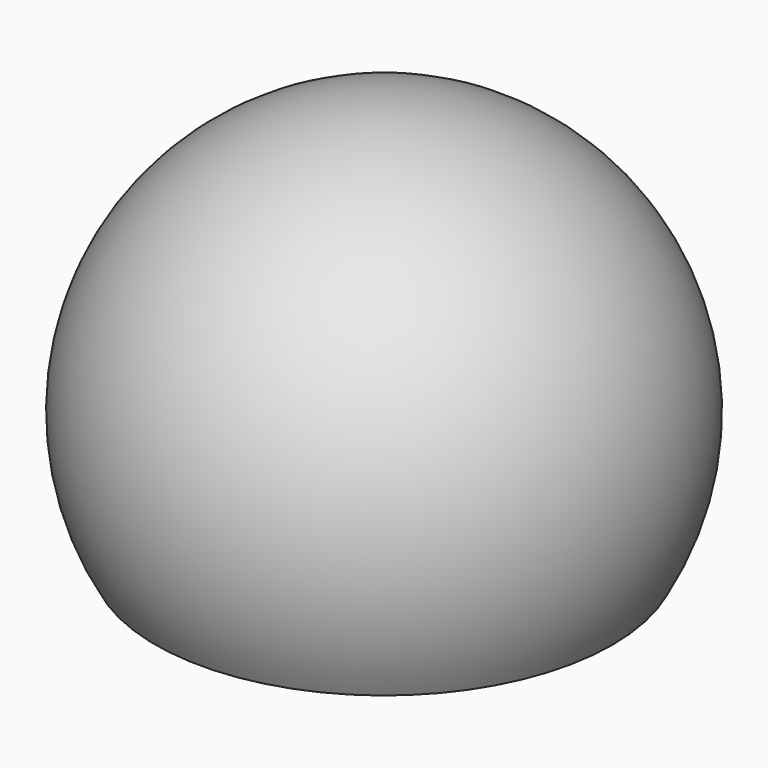
from build123d import *

# Parameters (mm, degrees)
F2_R = 1.19999
F3_R = 1.5


# Not quite as in the source:
# - a fillet or chamfer is up to 0.001 mm smaller than in the source, because OpenCascade refuses the exact size


with BuildPart() as f1:
    # F0 (on Front) → F1 (revolve)
    with BuildSketch(Plane.XZ):
        with BuildLine():
            Line((0, 22.8), (0, 24))
            ThreePointArc((0, 24), (-13.8564064606, 16), (-13.8564064606, 0))
            Line((-13.8564064606, 0), (-12.451505933, 0))
            ThreePointArc((-12.451505933, 0), (-13.8029789452, 13.3402033893), (-3.825, 22.2971806661))
            ThreePointArc((-3.825, 22.2971806661), (-3.227786159, 22.4437320839), (-2.625, 22.5653484339))
            ThreePointArc((-2.625, 22.5653484339), (-1.3177335047, 22.741220384), (0, 22.8))
        make_face()
        with BuildLine():
            Line((-2.625, 18.0653484339), (-2.625, 22.5653484339))
            ThreePointArc((-2.625, 22.5653484339), (-3.227786159, 22.4437320839), (-3.825, 22.2971806661))
            Line((-3.825, 22.2971806661), (-3.825, 18.0653484339))
            Line((-3.825, 18.0653484339), (-2.625, 18.0653484339))
        make_face()
    revolve(axis=Axis((0, 0, 23.4), (0, 0, 1)))

    # F2 (radius 1.2 in the source; OpenCascade refuses exactly that, so slightly less here)
    f2_edges = [f1.edges().sort_by_distance(p)[0] for p in [
        (2.625, 0, 18.065348),
    ]]
    fillet(f2_edges, radius=F2_R)

    # F3
    f3_edges = [f1.edges().sort_by_distance(p)[0] for p in [
        (3.825, 0, 22.297181),
    ]]
    fillet(f3_edges, radius=F3_R)


solid = f1.part
